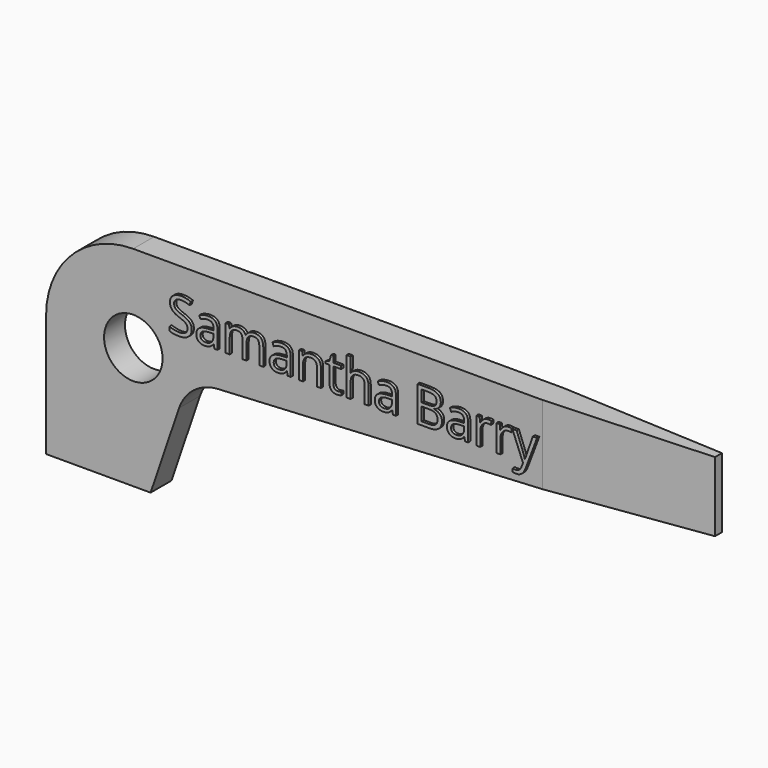
from build123d import *

# Parameters (mm, degrees)
F1_DEPTH     = 2.38125
F2_R         = 2.6655651251
F3_DEPTH     = 2.38225
F5_DEPTH     = 25.4
F6_TEXT_SIZE = 4.4906135687
F7_DEPTH     = 0.254


# Not quite as in the source:
# - Text() gives the source's letters only with a copy of the font that has no kerning and outlines rounded to 1/6400 em; it was checked with that copy


with BuildPart() as f1:
    # F0 (on Front) → F1 (new body)
    with BuildSketch(Plane.XZ):
        with BuildLine():
            Line((60.325, 19.05), (7.9375, 19.05))
            ThreePointArc((7.9375, 19.05), (2.3248399243, 16.7251600757), (0, 11.1125))
            Line((0, 11.1125), (0, 0))
            Line((0, 0), (9.525, 0))
            Line((9.525, 0), (12.1173647876, 7.6271664624))
            ThreePointArc((12.1173647876, 7.6271664624), (13.4786145605, 9.5135918491), (15.6631963617, 10.3130942181))
            Line((15.6631963617, 10.3130942181), (60.325, 12.7))
            Line((60.325, 12.7), (60.325, 19.05))
        make_face()
    extrude(amount=F1_DEPTH)

    # F2 (on face) → F3 (cut, through all)
    with BuildSketch(Plane.XZ.offset(2.38125)):
        with Locations((7.9502, 11.0998)):
            Circle(F2_R)
    extrude(amount=-F3_DEPTH, mode=Mode.SUBTRACT)

    # F4 (on face) → F5 (cut)
    with BuildSketch(Plane.XY.offset(19.05)):
        Polygon((60.325, 0), (45.24375, 0), (60.325, -0.79375), align=None)
        Polygon((60.325, -2.38125), (60.325, -1.5875), (45.24375, -2.38125), align=None)
    extrude(amount=-F5_DEPTH, mode=Mode.SUBTRACT)

    # F6 (on face) → F7 (join)
    with BuildSketch(Plane.XZ.offset(2.38125)):
        with Locations((11.2224406084, 13.6041921424)):
            Text('Samantha Barry', F6_TEXT_SIZE, font='Open Sans', text_align=(TextAlign.LEFT, TextAlign.BOTTOM))
    extrude(amount=F7_DEPTH)


solid = f1.part
